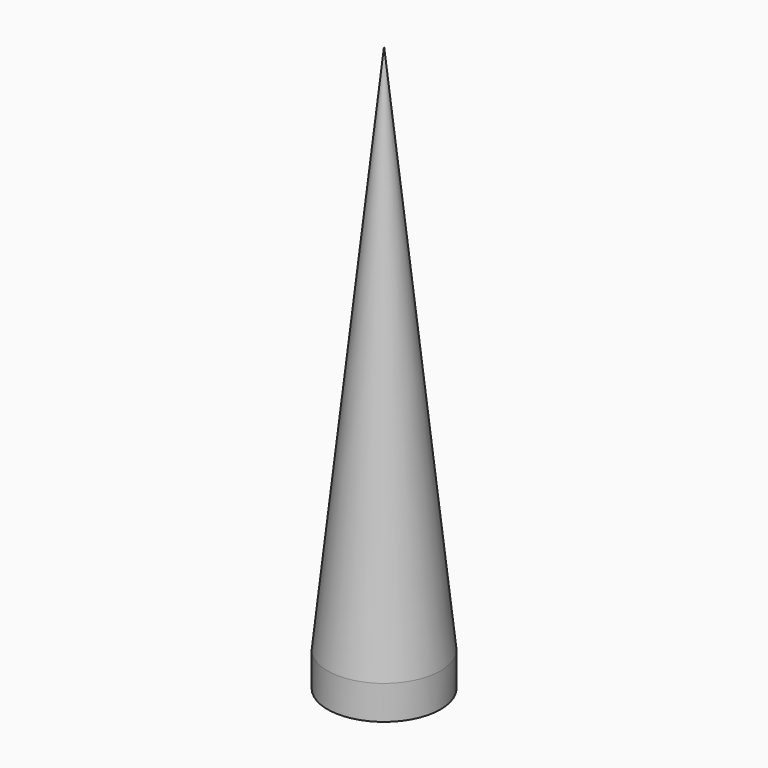
from build123d import *


# Not quite as in the source:
# - a feature of the source that left no trace in its solid (it failed there, or was rolled back) is left out
# - the program builds the solid bodies; features that only make, move or delete a surface that nothing else refers to are left out


with BuildPart() as f1:
    # F0 (on Front) → F1 (revolve)
    with BuildSketch(Plane.XZ):
        Polygon((5, -22.5757566782), (5, -19.5757566782), (0, 27.4242433218), (0, -22.5757566782), align=None)
    revolve(axis=Axis((0, 0, 2.4242433218), (0, 0, 1)))


solid = f1.part
